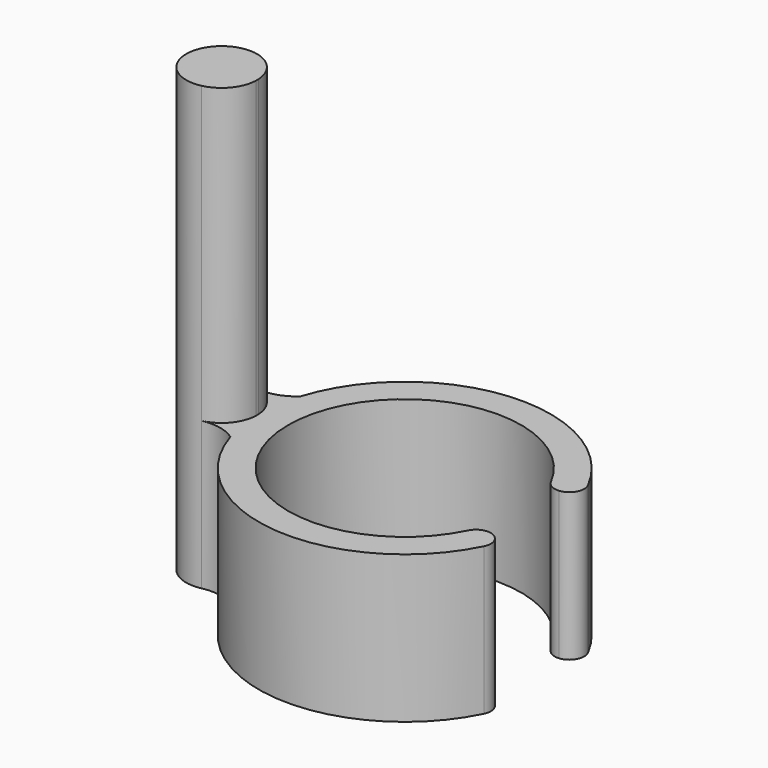
from build123d import *

# Parameters (mm, degrees)
F1_DEPTH = 10
F2_DEPTH = 30
F3_R     = 0.99999


# Not quite as in the source:
# - a fillet or chamfer is up to 0.001 mm smaller than in the source, because OpenCascade refuses the exact size


with BuildPart() as f1:
    # F0 (on Top) → F1 (new body)
    with BuildSketch(Plane.XY):
        with BuildLine():
            ThreePointArc((-9.4454545455, 2.9653648055), (-9.7857038582, 1.5), (-9.9, 0))
            ThreePointArc((-9.9, 0), (-9.896558825, -0.0741336209), (-9.895411401, -0.1483381952))
            ThreePointArc((-9.895411401, -0.1483381952), (-9.8958382083, -0.193598479), (-9.8971184787, -0.238842665))
            ThreePointArc((-9.8971184787, -0.238842665), (-9.7668963107, -1.6179420433), (-9.4454545455, -2.9653648055))
            ThreePointArc((-9.4454545455, -2.9653648055), (0.0988831148, -9.8995061558), (9.5028042321, -2.7760964907))
            Line((9.5028042321, -2.7760964907), (7.3082145562, -3))
            ThreePointArc((7.3082145562, -3), (-7.9, 0), (7.3082145562, 3))
            Line((7.3082145562, 3), (9.3680287257, 3.2015680213))
            ThreePointArc((9.3680287257, 3.2015680213), (-0.1242846699, 9.8992198339), (-9.4454545455, 2.9653648055))
        make_face()
        with BuildLine():
            ThreePointArc((-9.4454545455, 2.9653648055), (-10.6009515165, 2.3129966374), (-11.9248231248, 2.2228775962))
            ThreePointArc((-11.9248231248, 2.2228775962), (-10.5211552877, 1.4678348291), (-9.9, 0))
            ThreePointArc((-9.9, 0), (-9.7857038582, 1.5), (-9.4454545455, 2.9653648055))
        make_face()
        with BuildLine():
            ThreePointArc((-9.8971184787, -0.238842665), (-10.4571434039, -1.6913128454), (-11.7905485927, -2.4946360333))
            ThreePointArc((-11.7905485927, -2.4946360333), (-10.5690595937, -2.4861794722), (-9.4454545455, -2.9653648055))
            ThreePointArc((-9.4454545455, -2.9653648055), (-9.7668963107, -1.6179420433), (-9.8971184787, -0.238842665))
        make_face()
    extrude(amount=F1_DEPTH)

    # F0 (on Top) → F2 (join)
    with BuildSketch(Plane.XY):
        with BuildLine():
            ThreePointArc((-9.9, 0), (-10.5211552877, 1.4678348291), (-11.9248231248, 2.2228775962))
            ThreePointArc((-11.9248231248, 2.2228775962), (-14.6944398213, -0.2166217115), (-11.7905485927, -2.4946360333))
            ThreePointArc((-11.7905485927, -2.4946360333), (-10.4571434039, -1.6913128454), (-9.8971184787, -0.238842665))
            ThreePointArc((-9.8971184787, -0.238842665), (-9.8992795935, -0.1194300232), (-9.9, 0))
        make_face()
    extrude(amount=F2_DEPTH)

    # F3 (radius 1 in the source; OpenCascade refuses exactly that, so slightly less here)
    f3_edges = [f1.edges().sort_by_distance(p)[0] for p in [
        (9.502804, -2.776096, 5),
        (7.308215, -3, 5),
        (9.368029, 3.201568, 5),
        (7.308215, 3, 5),
    ]]
    fillet(f3_edges, radius=F3_R)


solid = f1.part
